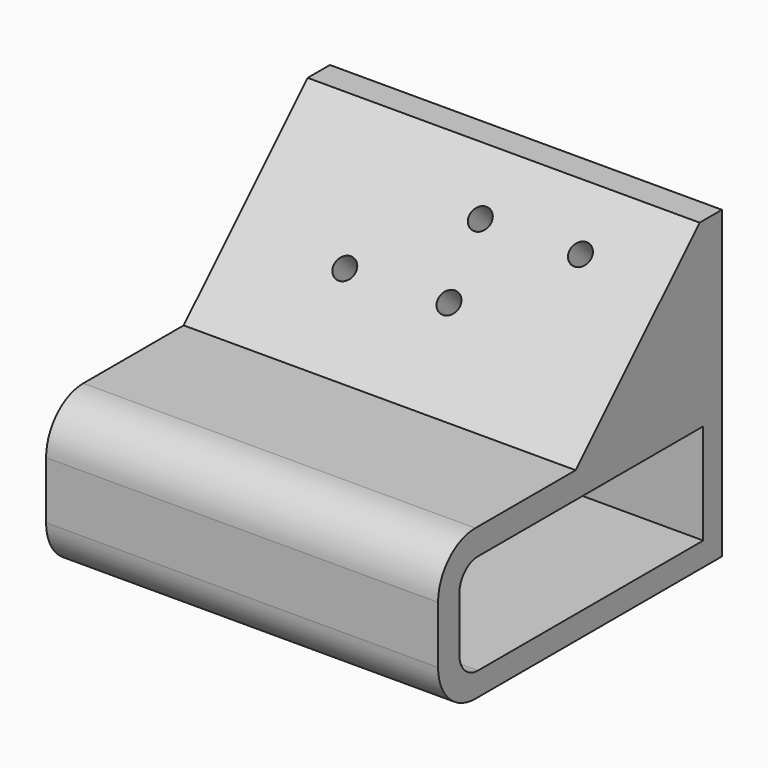
from build123d import *

# Parameters (mm, degrees)
F0_W        = 29.972
F0_H        = 50.038
F1_DEPTH    = 64.262
F2_SIZE     = 25.4
F3_DEPTH    = 28.194
F4_T1_DEPTH = 102.362
F5_R        = 1.7813508629
F6_DEPTH    = 12.192
F7_W        = 49.9822117854
F7_H        = 16.4834968746
F8_DEPTH    = 137.16
F9_R        = 3.81


# Not quite as in the source:
# - a fillet or chamfer that OpenCascade refuses, or shapes differently, is made with other operations: its cross-section is extruded or revolved along the edge and cut away or added


with BuildPart() as f1:
    # F0 (on Right) → F1 (new body)
    with BuildSketch(Plane.YZ):
        with Locations((-12.6866316661, -8.6694222925)):
            Rectangle(F0_W, F0_H)
    extrude(amount=F1_DEPTH)

    # F2
    f2_edges = [f1.edges().sort_by_distance(p)[0] for p in [
        (32.131, -27.672632, 16.349578),
    ]]
    chamfer(f2_edges, length=F2_SIZE)

    # F3 (add): a face of the model
    f3_faces = [f1.faces().sort_by_distance(p)[0] for p in [
        (32.131, -27.6726316661, -21.3694222925),
    ]]
    extrude(f3_faces, amount=F3_DEPTH)

    # F4: fillet of radius 7.62 on 4 edges, made by hand

    # F4_s2 → F4_t1 (cut)
    with BuildSketch(Plane.YZ.offset(-19.05)):
        with BuildLine():
            ThreePointArc((-48.2466316661, -33.6884222925), (-53.6347853387, -31.4565759651), (-55.8666316661, -26.0684222925))
            Line((-55.8666316661, -26.0684222925), (-55.8666316661, -33.6884222925))
            Line((-55.8666316661, -33.6884222925), (-48.2466316661, -33.6884222925))
        make_face()
        with BuildLine():
            ThreePointArc((-55.8666316661, -16.6704222925), (-53.6347853387, -11.2822686198), (-48.2466316661, -9.0504222925))
            Line((-48.2466316661, -9.0504222925), (-55.8666316661, -9.0504222925))
            Line((-55.8666316661, -9.0504222925), (-55.8666316661, -16.6704222925))
        make_face()
    extrude(amount=F4_T1_DEPTH, mode=Mode.SUBTRACT)

    # F5 (on face) → F6 (cut)
    with BuildSketch(Plane(origin=(0, -9.3111046868, 9.3111046868), x_dir=(1, 0, 0), z_dir=(0, -0.7071067812, 0.7071067812))):
        with Locations((35.1360822096, -11.1896051094)):
            Circle(F5_R)
        with Locations((49.9720936641, 0.6819777191)):
            Circle(F5_R)
        with Locations((33.6671667174, 0.486287754)):
            Circle(F5_R)
        with Locations((18.350715749, -11.7116672918)):
            Circle(F5_R)
    extrude(amount=-F6_DEPTH, mode=Mode.SUBTRACT)

    # F7 (on face) → F8 (cut)
    with BuildSketch(Plane.YZ.offset(64.262)):
        with Locations((-26.5206474578, -21.5896144509)):
            Rectangle(F7_W, F7_H)
    extrude(amount=-F8_DEPTH, mode=Mode.SUBTRACT)

    # F9
    f9_edges = [f1.edges().sort_by_distance(p)[0] for p in [
        (32.131, -51.511753, -13.347866),
        (32.131, -51.511753, -29.831363),
    ]]
    fillet(f9_edges, radius=F9_R)


solid = f1.part
